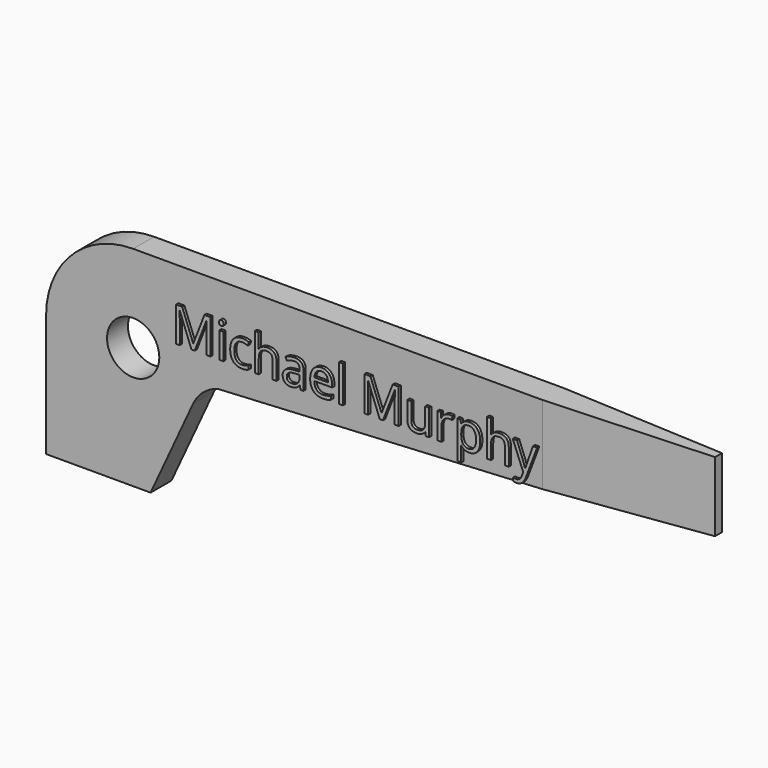
from build123d import *

# Parameters (mm, degrees)
F1_DEPTH     = 2.38125
F2_R         = 2.38125
F3_DEPTH     = 25.4
F5_DEPTH     = 25.4
F6_TEXT_SIZE = 4.4274165862
F7_DEPTH     = 0.254


# Not quite as in the source:
# - Text() gives the source's letters only with a copy of the font that has no kerning and outlines rounded to 1/6400 em; it was checked with that copy


with BuildPart() as f1:
    # F0 (on Front) → F1 (new body)
    with BuildSketch(Plane.XZ):
        with BuildLine():
            Line((60.325, 19.05), (7.9375, 19.05))
            ThreePointArc((7.9375, 19.05), (2.3248399243, 16.7251600757), (0, 11.1125))
            Line((0, 11.1125), (0, 0))
            Line((0, 0), (9.525, 0))
            Line((9.525, 0), (13.4001548854, 8.3972573633))
            ThreePointArc((13.4001548854, 8.3972573633), (14.3197174508, 9.6080595978), (15.6634210502, 10.3194652484))
            Line((15.6634210502, 10.3194652484), (60.325, 12.7))
            Line((60.325, 12.7), (60.325, 19.05))
        make_face()
    extrude(amount=F1_DEPTH)

    # F2 (on face) → F3 (cut)
    with BuildSketch(Plane.XZ.offset(2.38125)):
        with Locations((7.9375, 11.1125)):
            Circle(F2_R)
    extrude(amount=-F3_DEPTH, mode=Mode.SUBTRACT)

    # F4 (on face) → F5 (cut)
    with BuildSketch(Plane.XY.offset(19.05)):
        Polygon((60.325, 0), (45.24375, 0), (60.325, -0.79375), align=None)
        Polygon((60.325, -2.38125), (60.325, -1.5875), (45.24375, -2.38125), align=None)
    extrude(amount=-F5_DEPTH, mode=Mode.SUBTRACT)

    # F6 (on face) → F7 (join)
    with BuildSketch(Plane.XZ.offset(2.38125)):
        with Locations((11.6182128118, 12.8630206922)):
            Text('Michael Murphy', F6_TEXT_SIZE, font='Open Sans', text_align=(TextAlign.LEFT, TextAlign.BOTTOM))
    extrude(amount=F7_DEPTH)


solid = f1.part
